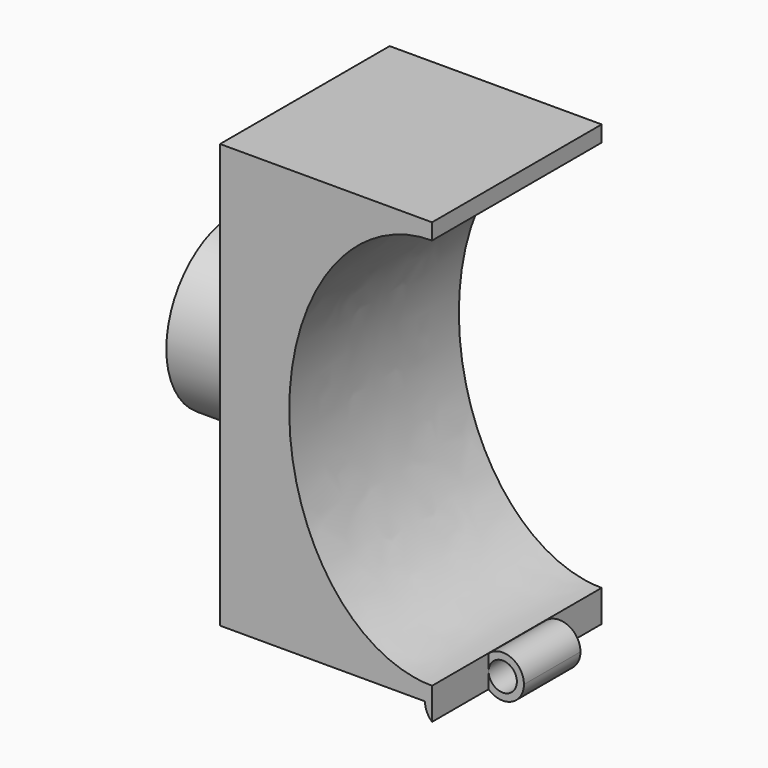
from build123d import *

# Parameters (mm, degrees)
F1_DEPTH  = 75
F2_R      = 30
F3_DEPTH  = 25
F4_R      = 5
F5_DEPTH  = 15
F7_DEPTH  = 75
F8_R      = 5
F9_DEPTH  = 75
F10_W     = 25
F10_H     = 45.2830219137
F10_W_2   = 34.9056578674
F10_H_2   = 56.6037699187
F11_DEPTH = 25


# Not quite as in the source:
# - a feature names something its author has since deleted; it is built from what else it names


with BuildPart() as f1:
    # F0 (on Front) → F1 (new body)
    with BuildSketch(Plane.XZ):
        with BuildLine():
            Line((-75, -75), (0, -75))
            Line((0, -75), (0, -69.3261250854))
            add(Edge.make_bspline(
                [(0, 69.3261250854), (-50.5212285231, 69.3261250854), (-50.5212285231, 0), (-50.5212285231, -69.3261250854), (0, -69.3261250854)],
                knots=[3.1415926536, 3.1415926536, 3.1415926536, 4.7123889804, 4.7123889804, 6.2831853072, 6.2831853072, 6.2831853072], degree=2, weights=[1, 0.7071067812, 1, 0.7071067812, 1]))
            Line((0, 69.3261250854), (0, 75))
            Line((0, 75), (-75, 75))
            Line((-75, 75), (-75, -75))
        make_face()
    extrude(amount=F1_DEPTH)

    # F2 (on face) → F3 (join)
    with BuildSketch(Plane(origin=(-75, 0, 0), x_dir=(0, -1, 0), z_dir=(-1, 0, 0))):
        with Locations((37.5, 0)):
            Circle(F2_R)
    extrude(amount=F3_DEPTH)

    # F4 (on face) → F5 (join)
    with BuildSketch(Plane(origin=(-100, 0, 0), x_dir=(0, -1, 0), z_dir=(-1, 0, 0))):
        with Locations((37.5, 0)):
            Circle(F4_R)
    extrude(amount=F5_DEPTH)

    # F6 (on face) → F7 (join)
    with BuildSketch(Plane.XZ.offset(75)):
        with BuildLine():
            ThreePointArc((-2.5, -75), (5, -82.5), (12.5, -75))
            ThreePointArc((12.5, -75), (8.0618621785, -68.1534680312), (0, -69.4098300563))
            Line((0, -69.4098300563), (0, -75))
            Line((0, -75), (-2.5, -75))
        make_face()
    extrude(amount=-F7_DEPTH)

    # F8 (on face) → F9 (cut)
    with BuildSketch(Plane.XZ.offset(75)):
        with Locations((5, -75)):
            Circle(F8_R)
    extrude(amount=-F9_DEPTH, mode=Mode.SUBTRACT)

    # F10 (on Right) → F11 (cut)
    with BuildSketch(Plane.YZ):
        with Locations((-62.5, -78.4633336838)):
            Rectangle(F10_W, F10_H)
        with Locations((-7.5471710663, -85.2243384972)):
            Rectangle(F10_W_2, F10_H_2)
    extrude(amount=F11_DEPTH, mode=Mode.SUBTRACT)


solid = f1.part
